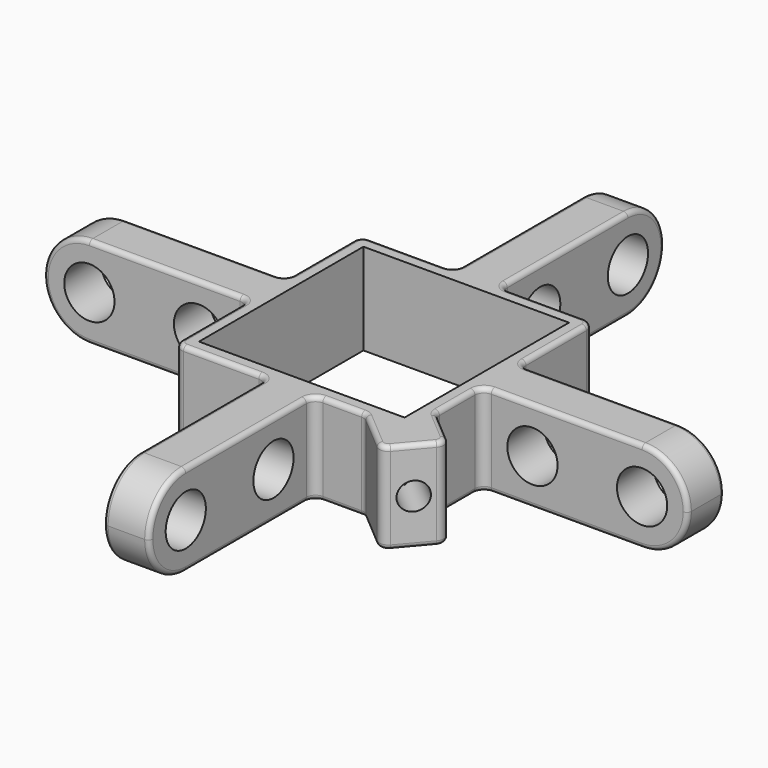
from build123d import *

# Parameters (mm, degrees)
F0_W     = 10
F0_H     = 45
F0_W_2   = 45
F0_H_2   = 10
F1_DEPTH = 20
F2_R     = 5.5
F3_DEPTH = 10
F4_R     = 5.5
F5_DEPTH = 10
F6_R     = 9.99999
F7_R     = 3
F8_DEPTH = 25
F9_R     = 2
F10_R    = 1


# Not quite as in the source:
# - a fillet or chamfer is up to 0.001 mm smaller than in the source, because OpenCascade refuses the exact size


with BuildPart() as f1:
    # F0 (on Top) → F1 (new body)
    with BuildSketch(Plane.XY):
        with Locations((0, 48)):
            Rectangle(F0_W, F0_H)
        with Locations((-48, 0)):
            Rectangle(F0_W_2, F0_H_2)
        with Locations((0, -48)):
            Rectangle(F0_W, F0_H)
        with Locations((48, 0)):
            Rectangle(F0_W_2, F0_H_2)
        Polygon((5, 25.5), (-5, 25.5), (-25.5, 25.5), (-25.5, 5), (-25.5, -5), (-25.5, -25.5), (-5, -25.5), (5, -25.5), (16.2398189751, -25.5), (25.5, -25.5), (25.5, -17.6228334755), (25.5, -5), (25.5, 5), (25.5, 25.5), align=None)
        Rectangle(F0_W_2, F0_H, mode=Mode.SUBTRACT)
        Polygon((33.7834382075, -24.6691344042), (25.5, -17.6228334755), (25.5, -25.5), (16.2398189751, -25.5), (26.0082122366, -33.8094769088), align=None)
    extrude(amount=F1_DEPTH)

    # F2 (on face) → F3 (cut)
    with BuildSketch(Plane.XZ.offset(5)):
        with Locations((36.5, 10)):
            Circle(F2_R)
        with Locations((60.5, 10)):
            Circle(F2_R)
        with Locations((-36.5, 10)):
            Circle(F2_R)
        with Locations((-60.5, 10)):
            Circle(F2_R)
    extrude(amount=-F3_DEPTH, mode=Mode.SUBTRACT)

    # F4 (on face) → F5 (cut)
    with BuildSketch(Plane(origin=(-5, 0, 0), x_dir=(0, -1, 0), z_dir=(-1, 0, 0))):
        with Locations((36.5, 10)):
            Circle(F4_R)
        with Locations((60.5, 10)):
            Circle(F4_R)
        with Locations((-36.5, 10)):
            Circle(F4_R)
        with Locations((-60.5, 10)):
            Circle(F4_R)
    extrude(amount=-F5_DEPTH, mode=Mode.SUBTRACT)

    # F6 (radius 10 in the source; OpenCascade refuses exactly that, so slightly less here)
    f6_edges = [f1.edges().sort_by_distance(p)[0] for p in [
        (0, 70.5, 20),
        (0, 70.5, 0),
        (-70.5, 0, 0),
        (0, -70.5, 20),
        (70.5, 0, 20),
        (-70.5, 0, 20),
        (0, -70.5, 0),
        (70.5, 0, 0),
    ]]
    fillet(f6_edges, radius=F6_R)

    # F7 (on face) → F8 (cut)
    with BuildSketch(Plane(origin=(31.7754035757, -27.02972487, 0), x_dir=(0.6479354976, 0.7616952087, 0), z_dir=(0.7616952087, -0.6479354976, 0))):
        with Locations((-2.9008726342, 10)):
            Circle(F7_R)
    extrude(amount=-F8_DEPTH, mode=Mode.SUBTRACT)

    # F9
    f9_edges = [f1.edges().sort_by_distance(p)[0] for p in [
        (-25.5, -5, 10),
        (-5, -25.5, 10),
        (16.239819, -25.5, 10),
        (5, -25.5, 10),
        (-5, 25.5, 10),
        (-25.5, 5, 10),
        (5, 25.5, 10),
        (25.5, 5, 10),
        (25.5, -17.622833, 10),
        (25.5, -5, 10),
        (-25.5, -25.5, 10),
        (25.5, 25.5, 10),
        (-25.5, 25.5, 10),
        (26.008212, -33.809477, 10),
        (33.783438, -24.669134, 10),
    ]]
    fillet(f9_edges, radius=F9_R)

    # F10
    f10_edges = [f1.edges().sort_by_distance(p)[0] for p in [
        (-15.25, 25.5, 20),
        (-25.5, 15.25, 20),
        (-25.5, -15.25, 20),
        (-15.25, -25.5, 20),
        (11.252119, -25.5, 20),
        (29.895825, -29.239306, 20),
        (25.5, -11.849205, 20),
        (25.5, 15.25, 20),
        (15.25, 25.5, 20),
        (24.484822, -32.513606, 10),
        (32.260048, -23.373263, 10),
    ]]
    fillet(f10_edges, radius=F10_R)


solid = f1.part
